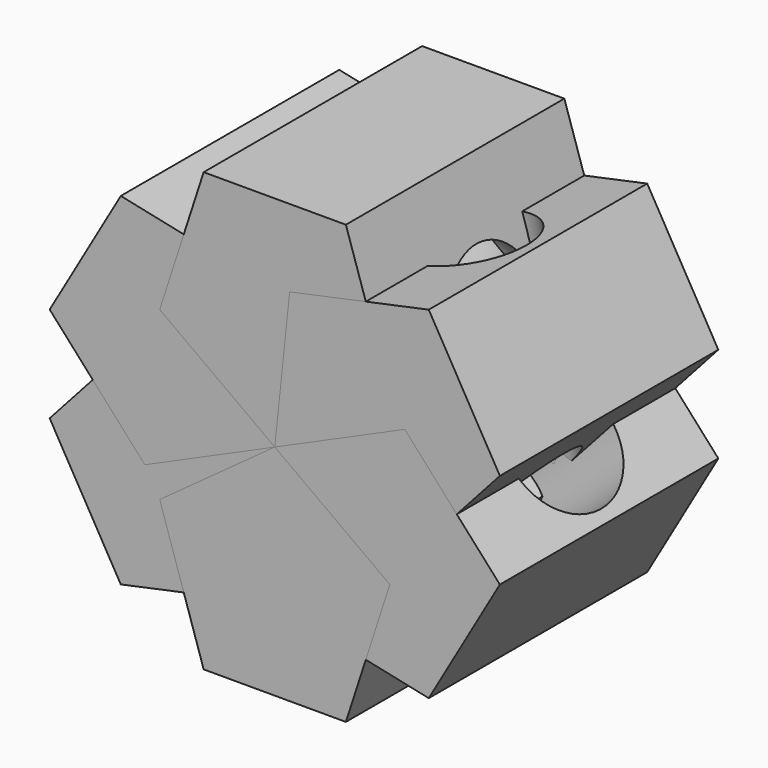
from build123d import *

# Parameters (mm, degrees)
F1_DEPTH = 184.6079975367
F2_R     = 40.1781170216
F3_DEPTH = 147.9660815238
F4_COUNT = 6
F5_R     = 38.8529332232
F6_DEPTH = 50.8


with BuildPart() as f1:
    # F0 (on Front) → F1 (new body)
    with BuildSketch(Plane.XZ):
        Polygon((-48.0770942615, -66.1724433303), (48.0770942615, -66.1724433303), (77.7903725954, 25.2756242335), (0, 81.7936381935), (-77.7903725954, 25.2756242335), align=None)
    extrude(amount=F1_DEPTH)

    # F2 (on face) → F3 (cut, through all)
    with BuildSketch(Plane(origin=(62.9337334284, 0, -20.4484095484), x_dir=(0, 1, 0), z_dir=(0.9510565163, 0, -0.3090169944))):
        with Locations((-92.3039987683, 0)):
            Circle(F2_R)
    extrude(amount=-F3_DEPTH, mode=Mode.SUBTRACT)


with BuildPart() as f4_1:
    # F4: instance of F1
    add(f1.part.rotate(Axis((0, -92.3039987683, 81.7936381935), (0, 1, 0)), 1 * 360 / F4_COUNT))


with BuildPart() as f4_2:
    # F4: instance of F1
    add(f1.part.rotate(Axis((0, -92.3039987683, 81.7936381935), (0, 1, 0)), 2 * 360 / F4_COUNT))


with BuildPart() as f4_3:
    # F4: instance of F1
    add(f1.part.rotate(Axis((0, -92.3039987683, 81.7936381935), (0, 1, 0)), 3 * 360 / F4_COUNT))


with BuildPart() as f4_4:
    # F4: instance of F1
    add(f1.part.rotate(Axis((0, -92.3039987683, 81.7936381935), (0, 1, 0)), 4 * 360 / F4_COUNT))


with BuildPart() as f4_5:
    # F4: instance of F1
    add(f1.part.rotate(Axis((0, -92.3039987683, 81.7936381935), (0, 1, 0)), 5 * 360 / F4_COUNT))


with BuildPart() as f1_1:
    add(f1.part)

    # F5 (on face) → F6 (cut)
    with BuildSketch(Plane(origin=(0, 0, -66.1724433303), x_dir=(1, 0, 0), z_dir=(0, 0, -1))):
        with Locations((0, 73.9705562592)):
            Circle(F5_R)
    extrude(amount=-F6_DEPTH, mode=Mode.SUBTRACT)


solid = Compound([f4_1.part, f4_2.part, f4_3.part, f4_4.part, f4_5.part, f1_1.part])
